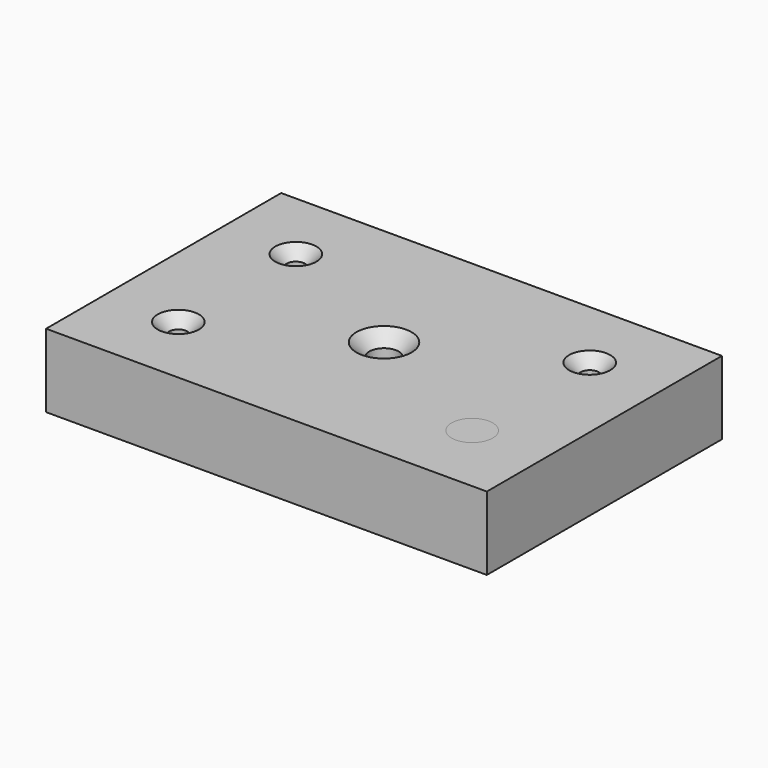
from build123d import *

# Parameters (mm, degrees)
F0_W           = 120
F0_H           = 80
F1_DEPTH       = 20
F3_D           = 5
F3_DEPTH       = 12
F3_CSINK_D     = 11.2
F3_CSINK_ANGLE = 90
F3_TIP         = 1.5021515476
F4_R           = 5.6
F5_DEPTH       = 20
F8_D           = 8
F8_DEPTH       = 12
F8_CSINK_D     = 15
F8_CSINK_ANGLE = 90
F8_TIP         = 2.4034424761


with BuildPart() as f1:
    # F0 (on Top) → F1 (new body)
    with BuildSketch(Plane.XY):
        Rectangle(F0_W, F0_H)
    extrude(amount=F1_DEPTH)

    # F3
    with Locations(Plane.XY.offset(20)):
        with Locations((-40, -20), (40, -20), (40, 20), (-40, 20)):
            CounterSinkHole(F3_D / 2, F3_CSINK_D / 2, depth=F3_DEPTH, counter_sink_angle=F3_CSINK_ANGLE)
            with Locations((0, 0, -(F3_DEPTH + F3_TIP / 2))):  # 118° drill point
                Cone(0, F3_D / 2, F3_TIP, mode=Mode.SUBTRACT)


with BuildPart() as f5:
    # F4 (on face) → F5 (new body)
    with BuildSketch(Plane.XY.offset(20)):
        with Locations((40, -20)):
            Circle(F4_R)
    extrude(amount=-F5_DEPTH)

    # F6: cut F1
    add(f1.part, mode=Mode.SUBTRACT)


with BuildPart() as f1_1:
    add(f1.part)

    # F8
    with Locations(Plane.XY.offset(20)):
        with Locations((0, 0)):
            CounterSinkHole(F8_D / 2, F8_CSINK_D / 2, depth=F8_DEPTH, counter_sink_angle=F8_CSINK_ANGLE)
            with Locations((0, 0, -(F8_DEPTH + F8_TIP / 2))):  # 118° drill point
                Cone(0, F8_D / 2, F8_TIP, mode=Mode.SUBTRACT)


solid = Compound([f5.part, f1_1.part])
